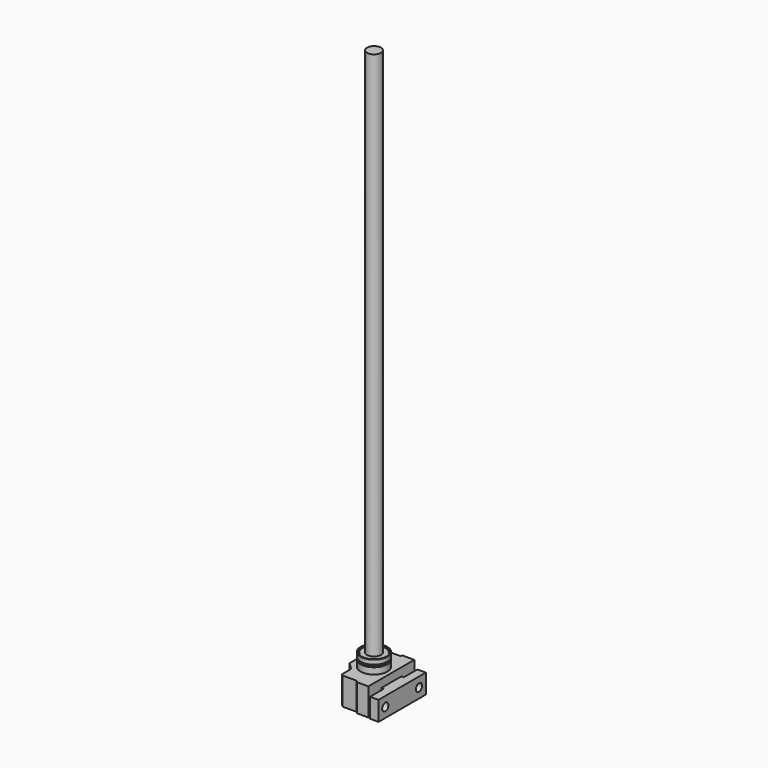
from build123d import *

# Parameters (mm, degrees)
F1_DEPTH  = 13.8
F2_R      = 2.75
F3_DEPTH  = 6.001
F4_R      = 9.5
F5_DEPTH  = 19.5
F4_R_2    = 8.25
F6_DEPTH  = 29
F7_START  = 0.5
F4_R_3    = 5
F7_DEPTH  = 28
F8_W      = 1
F8_H      = 1.25
F10_SIZE  = 0.2
F11_R     = 2.5
F12_DEPTH = 28.201
F13_DEPTH = 405


with BuildPart() as f1:
    # F0 (on Top) → F1 (new body)
    with BuildSketch(Plane.XY):
        with BuildLine():
            Line((20, -21), (20, 21))
            Line((20, 21), (14, 21))
            Line((14, 21), (14, 8.9))
            Line((14, 8.9), (-12.8, 8.9))
            Line((-12.8, 8.9), (-12.8, 0.5))
            Line((-12.8, 0.5), (-4.9749371855, 0.5))
            ThreePointArc((-4.9749371855, 0.5), (5, 0), (-4.9749371855, -0.5))
            Line((-4.9749371855, -0.5), (-12.8, -0.5))
            Line((-12.8, -0.5), (-12.8, -8.9))
            Line((-12.8, -8.9), (14, -8.9))
            Line((14, -8.9), (14, -21))
            Line((14, -21), (20, -21))
        make_face()
    extrude(amount=F1_DEPTH)

    # F2 (on face) → F3 (cut, through all)
    with BuildSketch(Plane(origin=(14, 0, 0), x_dir=(0, -1, 0), z_dir=(-1, 0, 0))):
        with Locations((-14.95, 6.9)):
            Circle(F2_R)
        with Locations((14.95, 6.9)):
            Circle(F2_R)
    extrude(amount=-F3_DEPTH, mode=Mode.SUBTRACT)


with BuildPart() as f5:
    # F4 (on Top) → F5 (new body)
    with BuildSketch(Plane.XY):
        Polygon((12.3, -20.4), (12.3, 20.4), (4.3, 20.4), (3.05, 19.15), (-7.05, 19.15), (-8.2, 18), (-8.2, 10), (-13.2, 5.25), (-13.2, -5.25), (-8.2, -10), (-8.2, -18), (-7.05, -19.15), (3.05, -19.15), (4.3, -20.4), align=None)
        Circle(F4_R, mode=Mode.SUBTRACT)
    extrude(amount=F5_DEPTH)

    # F11 (on face) → F12 (cut, through all)
    with BuildSketch(Plane(origin=(-8.2, 0, 0), x_dir=(0, -1, 0), z_dir=(-1, 0, 0))):
        with Locations((14, 9.75)):
            Circle(F11_R)
        with Locations((-14, 9.75)):
            Circle(F11_R)
    extrude(amount=-F12_DEPTH, mode=Mode.SUBTRACT)


with BuildPart() as f6:
    # F4 (on Top) → F6 (new body)
    with BuildSketch(Plane.XY):
        Circle(F4_R)
        Circle(F4_R_2, mode=Mode.SUBTRACT)
    extrude(amount=F6_DEPTH)

    # F4 (on Top) → F7 (join)
    with BuildSketch(Plane.XY.offset(F7_START)):
        Circle(F4_R_2)
        Circle(F4_R_3, mode=Mode.SUBTRACT)
    extrude(amount=F7_DEPTH)

    # F8 (on Front) → F9 (revolve, cut)
    with BuildSketch(Plane.XZ):
        with Locations((-9, 24.875)):
            Rectangle(F8_W, F8_H)
        with Locations((-9, 4.125)):
            Rectangle(F8_W, F8_H)
    revolve(axis=Axis((0, 0, 7.25), (0, 0, 1)), mode=Mode.SUBTRACT)

    # F10
    f10_edges = [f6.edges().sort_by_distance(p)[0] for p in [
        (-9.5, 0, 29),
        (-8.25, 0, 29),
        (-9.5, 0, 24.25),
        (-9.5, 0, 25.5),
        (-9.5, 0, 3.5),
        (-9.5, 0, 4.75),
        (-9.5, 0, 0),
        (-8.25, 0, 0),
    ]]
    chamfer(f10_edges, length=F10_SIZE)


with BuildPart() as f13:
    # F4 (on Top) → F13 (new body)
    with BuildSketch(Plane.XY):
        Circle(F4_R_3)
    extrude(amount=F13_DEPTH)


solid = Compound([f1.part, f5.part, f6.part, f13.part])
